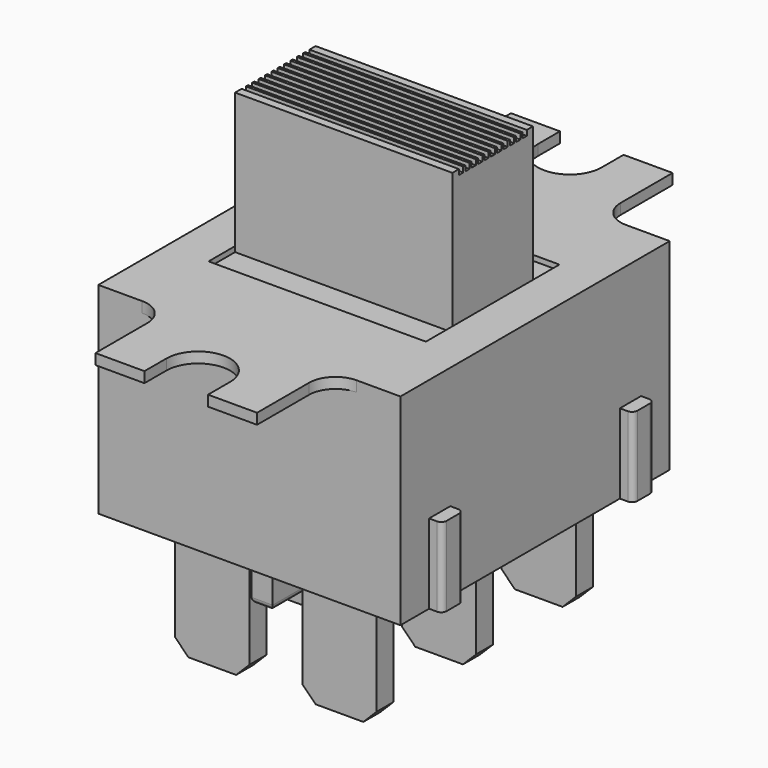
from build123d import *

# Parameters (mm, degrees)
F0_W      = 2.65
F0_H      = 12.7
F0_W_2    = 6.1
F0_H_2    = 3.45
F1_DEPTH  = 0.4
F2_W      = 2.4
F2_H      = 1.035
F3_DEPTH  = 1
F4_W      = 8.2
F4_H      = 6.3
F5_DEPTH  = 0.2
F6_W      = 8.2
F6_H      = 3.8
F7_DEPTH  = 5.3
F8_W      = 11.4
F8_H      = 12.7
F9_DEPTH  = 7.2
F10_W     = 1
F10_H     = 3
F11_DEPTH = 0.5
F12_W     = 2.8
F12_H     = 0.8
F13_DEPTH = 4.5
F14_R     = 1
F15_SIZE  = 0.5
F16_W     = 0.8
F16_H     = 11.5
F17_DEPTH = 1.5
F18_R     = 0.2
F19_W     = 0.2
F19_H     = 0.2
F20_DEPTH = 25


with BuildPart() as f1:
    # F0 (on Top) → F1 (new body)
    with BuildSketch(Plane.XY):
        with Locations((4.375, 0)):
            Rectangle(F0_W, F0_H)
        with Locations((0, -8.075)):
            Rectangle(F0_W_2, F0_H_2)
        Rectangle(F0_W_2, F0_H)
        with Locations((-4.375, 0)):
            Rectangle(F0_W, F0_H)
        with Locations((0, 8.075)):
            Rectangle(F0_W_2, F0_H_2)
    extrude(amount=F1_DEPTH)

    # F2 (on face) → F3 (cut)
    with BuildSketch(Plane.XY.offset(0.4)):
        with BuildLine():
            ThreePointArc((-1.2, 8.765), (0, 7.565), (1.2, 8.765))
            Line((1.2, 8.765), (-1.2, 8.765))
        make_face()
        with Locations((0, 9.2825)):
            Rectangle(F2_W, F2_H)
        with BuildLine():
            Line((-1.2, -8.765), (1.2, -8.765))
            ThreePointArc((1.2, -8.765), (0, -7.565), (-1.2, -8.765))
        make_face()
        with Locations((0, -9.2825)):
            Rectangle(F2_W, F2_H)
    extrude(amount=-F3_DEPTH, mode=Mode.SUBTRACT)

    # F4 (on face) → F5 (cut)
    with BuildSketch(Plane.XY.offset(0.4)):
        Rectangle(F4_W, F4_H)
    extrude(amount=-F5_DEPTH, mode=Mode.SUBTRACT)

    # F6 (on face) → F7 (join)
    with BuildSketch(Plane.XY.offset(0.2)):
        Rectangle(F6_W, F6_H)
    extrude(amount=F7_DEPTH)

    # F8 (on face) → F9 (join)
    with BuildSketch(Plane(origin=(0, 0, 0), x_dir=(1, 0, 0), z_dir=(0, 0, -1))):
        Rectangle(F8_W, F8_H)
    extrude(amount=F9_DEPTH)

    # F10 (on face) → F11 (join)
    with BuildSketch(Plane.YZ.offset(5.7)):
        with Locations((4.5, -5.7)):
            Rectangle(F10_W, F10_H)
        with Locations((-4.5, -5.7)):
            Rectangle(F10_W, F10_H)
    extrude(amount=F11_DEPTH)

    # F12 (on face) → F13 (join)
    with BuildSketch(Plane(origin=(0, 0, -7.2), x_dir=(1, 0, 0), z_dir=(0, 0, -1))):
        with Locations((2.4, -4.7)):
            Rectangle(F12_W, F12_H)
        with Locations((2.4, 0)):
            Rectangle(F12_W, F12_H)
        with Locations((2.4, 4.7)):
            Rectangle(F12_W, F12_H)
        with Locations((-2.4, -4.7)):
            Rectangle(F12_W, F12_H)
        with Locations((-2.4, 0)):
            Rectangle(F12_W, F12_H)
        with Locations((-2.4, 4.7)):
            Rectangle(F12_W, F12_H)
    extrude(amount=F13_DEPTH)

    # F14
    f14_edges = [f1.edges().sort_by_distance(p)[0] for p in [
        (3.05, 6.35, 0.2),
        (-3.05, 6.35, 0.2),
        (3.05, -6.35, 0.2),
        (-3.05, -6.35, 0.2),
    ]]
    fillet(f14_edges, radius=F14_R)

    # F15
    f15_edges = [f1.edges().sort_by_distance(p)[0] for p in [
        (1, 4.7, -11.7),
        (3.8, 4.7, -11.7),
        (-1, 4.7, -11.7),
        (-3.8, 4.7, -11.7),
        (1, 0, -11.7),
        (3.8, 0, -11.7),
        (-1, 0, -11.7),
        (-3.8, 0, -11.7),
        (-3.8, -4.7, -11.7),
        (-1, -4.7, -11.7),
        (1, -4.7, -11.7),
        (3.8, -4.7, -11.7),
    ]]
    chamfer(f15_edges, length=F15_SIZE)

    # F16 (on face) → F17 (join)
    with BuildSketch(Plane(origin=(0, 0, -7.2), x_dir=(1, 0, 0), z_dir=(0, 0, -1))):
        Rectangle(F16_W, F16_H)
    extrude(amount=F17_DEPTH)

    # F18
    f18_edges = [f1.edges().sort_by_distance(p)[0] for p in [
        (0, -5.75, -8.7),
        (0, 5.75, -8.7),
        (0.4, 0, -8.7),
        (-0.4, 0, -8.7),
        (6.2, -5, -5.7),
        (6.2, -4, -5.7),
        (6.2, 5, -5.7),
        (6.2, 4, -5.7),
    ]]
    fillet(f18_edges, radius=F18_R)

    # F19 (on face) → F20 (cut)
    with BuildSketch(Plane.YZ.offset(4.1)):
        with Locations((-1.4904041938, 5.4)):
            Rectangle(F19_W, F19_H)
        with Locations((-1.1904041938, 5.4)):
            Rectangle(F19_W, F19_H)
        with Locations((-0.8904041938, 5.4)):
            Rectangle(F19_W, F19_H)
        with Locations((-0.5904041938, 5.4)):
            Rectangle(F19_W, F19_H)
        with Locations((-0.2904041938, 5.4)):
            Rectangle(F19_W, F19_H)
        with Locations((0.0095958062, 5.4)):
            Rectangle(F19_W, F19_H)
        with Locations((0.3095958062, 5.4)):
            Rectangle(F19_W, F19_H)
        with Locations((0.6095958062, 5.4)):
            Rectangle(F19_W, F19_H)
        with Locations((0.9095958062, 5.4)):
            Rectangle(F19_W, F19_H)
        with Locations((1.2095958062, 5.4)):
            Rectangle(F19_W, F19_H)
        with Locations((1.5095958062, 5.4)):
            Rectangle(F19_W, F19_H)
    extrude(amount=-F20_DEPTH, mode=Mode.SUBTRACT)


solid = f1.part
